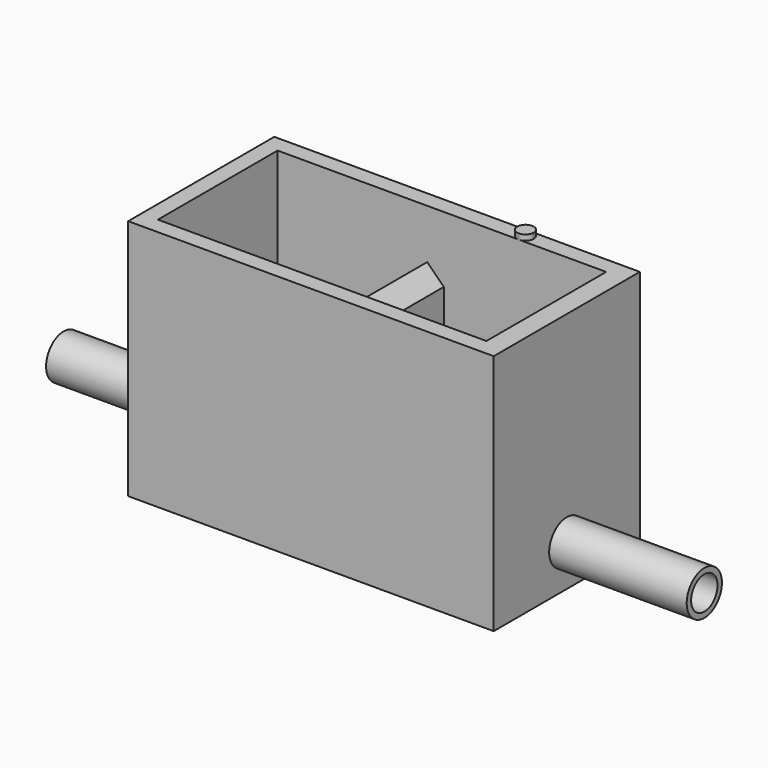
from build123d import *

# Parameters (mm, degrees)
F1_DEPTH     = 44
F0_W         = 27.2
F0_H         = 27.2
F2_DEPTH     = 1
F3_DEPTH     = 37
F4_R         = 4
F4_R_2       = 3
F5_DEPTH     = 25
F6_DEPTH     = 5
F7_R         = 4
F7_R_2       = 3
F8_DEPTH     = 25
F9_DEPTH     = 5
F10_T1_DEPTH = 27.2
F12_DEPTH    = 1


# Not quite as in the source:
# - a fillet or chamfer that OpenCascade refuses, or shapes differently, is made with other operations: its cross-section is extruded or revolved along the edge and cut away or added


with BuildPart() as f1:
    # F0 (on Top) → F1 (new body)
    with BuildSketch(Plane.XY):
        Polygon((49.8359054327, 16.6), (16.6, 16.6), (-16.6, 16.6), (-16.6, 3), (-16.6, 2), (-16.6, -2), (-16.6, -3), (-16.6, -16.6), (16.6, -16.6), (49.8359054327, -16.6), (49.8359054327, -3), (49.8359054327, -2), (49.8359054327, 2), (49.8359054327, 3), align=None)
        Polygon((16.6, -13.6), (13.6, -13.6), (-13.6, -13.6), (-13.6, 13.6), (13.6, 13.6), (16.6, 13.6), (46.1153909564, 13.6), (46.1153909564, -13.6), align=None, mode=Mode.SUBTRACT)
    extrude(amount=F1_DEPTH)

    # F0 (on Top) → F2 (join)
    with BuildSketch(Plane.XY):
        Rectangle(F0_W, F0_H)
        Polygon((16.6, -3), (16.6, -13.6), (46.1153909564, -13.6), (46.1153909564, 13.6), (16.6, 13.6), (16.6, 3), align=None)
    extrude(amount=F2_DEPTH)

    # F0 (on Top) → F3 (join)
    with BuildSketch(Plane.XY):
        Polygon((13.6, 13.6), (13.6, -13.6), (16.6, -13.6), (16.6, -3), (16.6, 3), (16.6, 13.6), align=None)
    extrude(amount=F3_DEPTH)

    # F4 (on face) → F5 (join)
    with BuildSketch(Plane(origin=(-16.6, 0, 0), x_dir=(0, -1, 0), z_dir=(-1, 0, 0))):
        with Locations((0, 7.5)):
            Circle(F4_R)
        with Locations((0, 7.5)):
            Circle(F4_R_2, mode=Mode.SUBTRACT)
    extrude(amount=F5_DEPTH)

    # F6 (cut): a face of the model
    f6_faces = [f1.faces().sort_by_distance(p)[0] for p in [
        (-16.6, 0, 7.5),
    ]]
    extrude(f6_faces, amount=-F6_DEPTH, mode=Mode.SUBTRACT)

    # F7 (on face) → F8 (join)
    with BuildSketch(Plane.YZ.offset(49.8359054327)):
        with Locations((0, 7.5)):
            Circle(F7_R)
        with Locations((0, 7.5)):
            Circle(F7_R_2, mode=Mode.SUBTRACT)
    extrude(amount=F8_DEPTH)

    # F9 (cut): a face of the model
    f9_faces = [f1.faces().sort_by_distance(p)[0] for p in [
        (49.8359054327, 0, 7.5),
    ]]
    extrude(f9_faces, amount=-F9_DEPTH, mode=Mode.SUBTRACT)

    # F10: chamfer of 5 on 1 edges, made by hand

    # F10_s2 → F10_t1 (cut)
    with BuildSketch(Plane.XZ.offset(-13.6)):
        Polygon((16.6, 32), (11.6, 37), (16.6, 37), align=None)
    extrude(amount=F10_T1_DEPTH, mode=Mode.SUBTRACT)

    # F11 (on face) → F12 (join)
    with BuildSketch(Plane.XY.offset(44)):
        with BuildLine():
            ThreePointArc((30.2547216209, 13.6), (31.315381806, 14.0393398209), (31.7547216415, 15.1))
            ThreePointArc((31.7547216415, 15.1), (31.3153818133, 16.1606601718), (30.2547216415, 16.6))
            ThreePointArc((30.2547216415, 16.6), (28.7547216415, 15.1000000103), (30.2547216209, 13.6))
        make_face()
    extrude(amount=F12_DEPTH)


solid = f1.part
